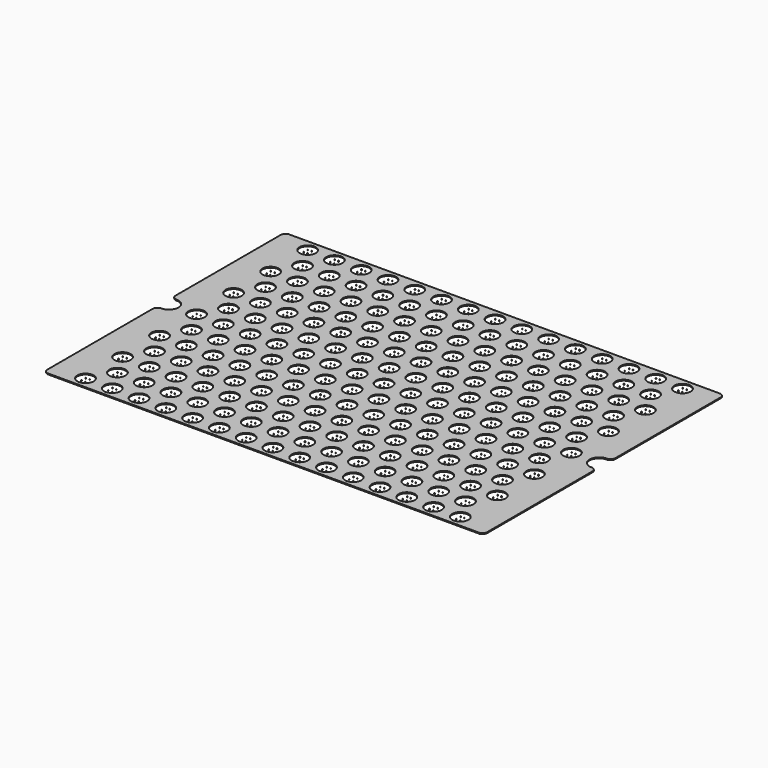
from build123d import *

# Parameters (mm, degrees)
F0_R     = 8.5
F1_DEPTH = 1
F2_R     = 0.25
F3_DEPTH = 1


with BuildPart() as f1:
    # F0 (on Top) → F1 (new body)
    with BuildSketch(Plane.XY):
        with BuildLine():
            Line((225, 157.5), (-225, 157.5))
            ThreePointArc((-225, 157.5), (-228.5355339059, 156.0355339059), (-230, 152.5))
            Line((-230, 152.5), (-230, 15))
            ThreePointArc((-230, 15), (-228.5355339059, 11.4644660941), (-225, 10))
            ThreePointArc((-225, 10), (-215, 0), (-225, -10))
            ThreePointArc((-225, -10), (-228.5355339059, -11.4644660941), (-230, -15))
            Line((-230, -15), (-230, -152.5))
            ThreePointArc((-230, -152.5), (-228.5355339059, -156.0355339059), (-225, -157.5))
            Line((-225, -157.5), (225, -157.5))
            ThreePointArc((225, -157.5), (228.5355339059, -156.0355339059), (230, -152.5))
            Line((230, -152.5), (230, -15))
            ThreePointArc((230, -15), (228.5355339059, -11.4644660941), (225, -10))
            ThreePointArc((225, -10), (215, 0), (225, 10))
            ThreePointArc((225, 10), (228.5355339059, 11.4644660941), (230, 15))
            Line((230, 15), (230, 152.5))
            ThreePointArc((230, 152.5), (228.5355339059, 156.0355339059), (225, 157.5))
        make_face()
        with Locations((-196, -145.2)):
            Circle(F0_R, mode=Mode.SUBTRACT)
        with Locations((-182, -121)):
            Circle(F0_R, mode=Mode.SUBTRACT)
        with Locations((-168, -145.2)):
            Circle(F0_R, mode=Mode.SUBTRACT)
        with Locations((-140, -145.2)):
            Circle(F0_R, mode=Mode.SUBTRACT)
        with Locations((-154, -121)):
            Circle(F0_R, mode=Mode.SUBTRACT)
        with Locations((-126, -121)):
            Circle(F0_R, mode=Mode.SUBTRACT)
        with Locations((-196, -96.8)):
            Circle(F0_R, mode=Mode.SUBTRACT)
        with Locations((-168, -96.8)):
            Circle(F0_R, mode=Mode.SUBTRACT)
        with Locations((-140, -96.8)):
            Circle(F0_R, mode=Mode.SUBTRACT)
        with Locations((-112, -145.2)):
            Circle(F0_R, mode=Mode.SUBTRACT)
        with Locations((-84, -145.2)):
            Circle(F0_R, mode=Mode.SUBTRACT)
        with Locations((-98, -121)):
            Circle(F0_R, mode=Mode.SUBTRACT)
        with Locations((-70, -121)):
            Circle(F0_R, mode=Mode.SUBTRACT)
        with Locations((-56, -145.2)):
            Circle(F0_R, mode=Mode.SUBTRACT)
        with Locations((-28, -145.2)):
            Circle(F0_R, mode=Mode.SUBTRACT)
        with Locations((-42, -121)):
            Circle(F0_R, mode=Mode.SUBTRACT)
        with Locations((-14, -121)):
            Circle(F0_R, mode=Mode.SUBTRACT)
        with Locations((-112, -96.8)):
            Circle(F0_R, mode=Mode.SUBTRACT)
        with Locations((-84, -96.8)):
            Circle(F0_R, mode=Mode.SUBTRACT)
        with Locations((-56, -96.8)):
            Circle(F0_R, mode=Mode.SUBTRACT)
        with Locations((-28, -96.8)):
            Circle(F0_R, mode=Mode.SUBTRACT)
        with Locations((-182, -72.6)):
            Circle(F0_R, mode=Mode.SUBTRACT)
        with Locations((-196, -48.4)):
            Circle(F0_R, mode=Mode.SUBTRACT)
        with Locations((-154, -72.6)):
            Circle(F0_R, mode=Mode.SUBTRACT)
        with Locations((-126, -72.6)):
            Circle(F0_R, mode=Mode.SUBTRACT)
        with Locations((-168, -48.4)):
            Circle(F0_R, mode=Mode.SUBTRACT)
        with Locations((-140, -48.4)):
            Circle(F0_R, mode=Mode.SUBTRACT)
        with Locations((-182, -24.2)):
            Circle(F0_R, mode=Mode.SUBTRACT)
        with Locations((-154, -24.2)):
            Circle(F0_R, mode=Mode.SUBTRACT)
        with Locations((-126, -24.2)):
            Circle(F0_R, mode=Mode.SUBTRACT)
        with Locations((-98, -72.6)):
            Circle(F0_R, mode=Mode.SUBTRACT)
        with Locations((-70, -72.6)):
            Circle(F0_R, mode=Mode.SUBTRACT)
        with Locations((-112, -48.4)):
            Circle(F0_R, mode=Mode.SUBTRACT)
        with Locations((-84, -48.4)):
            Circle(F0_R, mode=Mode.SUBTRACT)
        with Locations((-42, -72.6)):
            Circle(F0_R, mode=Mode.SUBTRACT)
        with Locations((-14, -72.6)):
            Circle(F0_R, mode=Mode.SUBTRACT)
        with Locations((-56, -48.4)):
            Circle(F0_R, mode=Mode.SUBTRACT)
        with Locations((-28, -48.4)):
            Circle(F0_R, mode=Mode.SUBTRACT)
        with Locations((-98, -24.2)):
            Circle(F0_R, mode=Mode.SUBTRACT)
        with Locations((-70, -24.2)):
            Circle(F0_R, mode=Mode.SUBTRACT)
        with Locations((-42, -24.2)):
            Circle(F0_R, mode=Mode.SUBTRACT)
        with Locations((-14, -24.2)):
            Circle(F0_R, mode=Mode.SUBTRACT)
        with Locations((0, -145.2)):
            Circle(F0_R, mode=Mode.SUBTRACT)
        with Locations((28, -145.2)):
            Circle(F0_R, mode=Mode.SUBTRACT)
        with Locations((56, -145.2)):
            Circle(F0_R, mode=Mode.SUBTRACT)
        with Locations((14, -121)):
            Circle(F0_R, mode=Mode.SUBTRACT)
        with Locations((42, -121)):
            Circle(F0_R, mode=Mode.SUBTRACT)
        with Locations((84, -145.2)):
            Circle(F0_R, mode=Mode.SUBTRACT)
        with Locations((112, -145.2)):
            Circle(F0_R, mode=Mode.SUBTRACT)
        with Locations((70, -121)):
            Circle(F0_R, mode=Mode.SUBTRACT)
        with Locations((98, -121)):
            Circle(F0_R, mode=Mode.SUBTRACT)
        with Locations((0, -96.8)):
            Circle(F0_R, mode=Mode.SUBTRACT)
        with Locations((28, -96.8)):
            Circle(F0_R, mode=Mode.SUBTRACT)
        with Locations((56, -96.8)):
            Circle(F0_R, mode=Mode.SUBTRACT)
        with Locations((84, -96.8)):
            Circle(F0_R, mode=Mode.SUBTRACT)
        with Locations((112, -96.8)):
            Circle(F0_R, mode=Mode.SUBTRACT)
        with Locations((140, -145.2)):
            Circle(F0_R, mode=Mode.SUBTRACT)
        with Locations((168, -145.2)):
            Circle(F0_R, mode=Mode.SUBTRACT)
        with Locations((126, -121)):
            Circle(F0_R, mode=Mode.SUBTRACT)
        with Locations((154, -121)):
            Circle(F0_R, mode=Mode.SUBTRACT)
        with Locations((196, -145.2)):
            Circle(F0_R, mode=Mode.SUBTRACT)
        with Locations((182, -121)):
            Circle(F0_R, mode=Mode.SUBTRACT)
        with Locations((140, -96.8)):
            Circle(F0_R, mode=Mode.SUBTRACT)
        with Locations((168, -96.8)):
            Circle(F0_R, mode=Mode.SUBTRACT)
        with Locations((196, -96.8)):
            Circle(F0_R, mode=Mode.SUBTRACT)
        with Locations((14, -72.6)):
            Circle(F0_R, mode=Mode.SUBTRACT)
        with Locations((42, -72.6)):
            Circle(F0_R, mode=Mode.SUBTRACT)
        with Locations((0, -48.4)):
            Circle(F0_R, mode=Mode.SUBTRACT)
        with Locations((28, -48.4)):
            Circle(F0_R, mode=Mode.SUBTRACT)
        with Locations((56, -48.4)):
            Circle(F0_R, mode=Mode.SUBTRACT)
        with Locations((70, -72.6)):
            Circle(F0_R, mode=Mode.SUBTRACT)
        with Locations((98, -72.6)):
            Circle(F0_R, mode=Mode.SUBTRACT)
        with Locations((84, -48.4)):
            Circle(F0_R, mode=Mode.SUBTRACT)
        with Locations((112, -48.4)):
            Circle(F0_R, mode=Mode.SUBTRACT)
        with Locations((14, -24.2)):
            Circle(F0_R, mode=Mode.SUBTRACT)
        with Locations((42, -24.2)):
            Circle(F0_R, mode=Mode.SUBTRACT)
        with Locations((70, -24.2)):
            Circle(F0_R, mode=Mode.SUBTRACT)
        with Locations((98, -24.2)):
            Circle(F0_R, mode=Mode.SUBTRACT)
        with Locations((126, -72.6)):
            Circle(F0_R, mode=Mode.SUBTRACT)
        with Locations((154, -72.6)):
            Circle(F0_R, mode=Mode.SUBTRACT)
        with Locations((140, -48.4)):
            Circle(F0_R, mode=Mode.SUBTRACT)
        with Locations((168, -48.4)):
            Circle(F0_R, mode=Mode.SUBTRACT)
        with Locations((182, -72.6)):
            Circle(F0_R, mode=Mode.SUBTRACT)
        with Locations((196, -48.4)):
            Circle(F0_R, mode=Mode.SUBTRACT)
        with Locations((126, -24.2)):
            Circle(F0_R, mode=Mode.SUBTRACT)
        with Locations((154, -24.2)):
            Circle(F0_R, mode=Mode.SUBTRACT)
        with Locations((182, -24.2)):
            Circle(F0_R, mode=Mode.SUBTRACT)
        with Locations((-196, 0)):
            Circle(F0_R, mode=Mode.SUBTRACT)
        with Locations((-182, 24.2)):
            Circle(F0_R, mode=Mode.SUBTRACT)
        with Locations((-168, 0)):
            Circle(F0_R, mode=Mode.SUBTRACT)
        with Locations((-140, 0)):
            Circle(F0_R, mode=Mode.SUBTRACT)
        with Locations((-154, 24.2)):
            Circle(F0_R, mode=Mode.SUBTRACT)
        with Locations((-126, 24.2)):
            Circle(F0_R, mode=Mode.SUBTRACT)
        with Locations((-196, 48.4)):
            Circle(F0_R, mode=Mode.SUBTRACT)
        with Locations((-182, 72.6)):
            Circle(F0_R, mode=Mode.SUBTRACT)
        with Locations((-168, 48.4)):
            Circle(F0_R, mode=Mode.SUBTRACT)
        with Locations((-140, 48.4)):
            Circle(F0_R, mode=Mode.SUBTRACT)
        with Locations((-154, 72.6)):
            Circle(F0_R, mode=Mode.SUBTRACT)
        with Locations((-126, 72.6)):
            Circle(F0_R, mode=Mode.SUBTRACT)
        with Locations((-112, 0)):
            Circle(F0_R, mode=Mode.SUBTRACT)
        with Locations((-84, 0)):
            Circle(F0_R, mode=Mode.SUBTRACT)
        with Locations((-98, 24.2)):
            Circle(F0_R, mode=Mode.SUBTRACT)
        with Locations((-70, 24.2)):
            Circle(F0_R, mode=Mode.SUBTRACT)
        with Locations((-56, 0)):
            Circle(F0_R, mode=Mode.SUBTRACT)
        with Locations((-28, 0)):
            Circle(F0_R, mode=Mode.SUBTRACT)
        with Locations((-42, 24.2)):
            Circle(F0_R, mode=Mode.SUBTRACT)
        with Locations((-14, 24.2)):
            Circle(F0_R, mode=Mode.SUBTRACT)
        with Locations((-112, 48.4)):
            Circle(F0_R, mode=Mode.SUBTRACT)
        with Locations((-84, 48.4)):
            Circle(F0_R, mode=Mode.SUBTRACT)
        with Locations((-98, 72.6)):
            Circle(F0_R, mode=Mode.SUBTRACT)
        with Locations((-70, 72.6)):
            Circle(F0_R, mode=Mode.SUBTRACT)
        with Locations((-56, 48.4)):
            Circle(F0_R, mode=Mode.SUBTRACT)
        with Locations((-28, 48.4)):
            Circle(F0_R, mode=Mode.SUBTRACT)
        with Locations((-42, 72.6)):
            Circle(F0_R, mode=Mode.SUBTRACT)
        with Locations((-14, 72.6)):
            Circle(F0_R, mode=Mode.SUBTRACT)
        with Locations((-196, 96.8)):
            Circle(F0_R, mode=Mode.SUBTRACT)
        with Locations((-168, 96.8)):
            Circle(F0_R, mode=Mode.SUBTRACT)
        with Locations((-140, 96.8)):
            Circle(F0_R, mode=Mode.SUBTRACT)
        with Locations((-182, 121)):
            Circle(F0_R, mode=Mode.SUBTRACT)
        with Locations((-196, 145.2)):
            Circle(F0_R, mode=Mode.SUBTRACT)
        with Locations((-154, 121)):
            Circle(F0_R, mode=Mode.SUBTRACT)
        with Locations((-126, 121)):
            Circle(F0_R, mode=Mode.SUBTRACT)
        with Locations((-168, 145.2)):
            Circle(F0_R, mode=Mode.SUBTRACT)
        with Locations((-140, 145.2)):
            Circle(F0_R, mode=Mode.SUBTRACT)
        with Locations((-112, 96.8)):
            Circle(F0_R, mode=Mode.SUBTRACT)
        with Locations((-84, 96.8)):
            Circle(F0_R, mode=Mode.SUBTRACT)
        with Locations((-56, 96.8)):
            Circle(F0_R, mode=Mode.SUBTRACT)
        with Locations((-28, 96.8)):
            Circle(F0_R, mode=Mode.SUBTRACT)
        with Locations((-98, 121)):
            Circle(F0_R, mode=Mode.SUBTRACT)
        with Locations((-70, 121)):
            Circle(F0_R, mode=Mode.SUBTRACT)
        with Locations((-112, 145.2)):
            Circle(F0_R, mode=Mode.SUBTRACT)
        with Locations((-84, 145.2)):
            Circle(F0_R, mode=Mode.SUBTRACT)
        with Locations((-42, 121)):
            Circle(F0_R, mode=Mode.SUBTRACT)
        with Locations((-14, 121)):
            Circle(F0_R, mode=Mode.SUBTRACT)
        with Locations((-56, 145.2)):
            Circle(F0_R, mode=Mode.SUBTRACT)
        with Locations((-28, 145.2)):
            Circle(F0_R, mode=Mode.SUBTRACT)
        Circle(F0_R, mode=Mode.SUBTRACT)
        with Locations((28, 0)):
            Circle(F0_R, mode=Mode.SUBTRACT)
        with Locations((56, 0)):
            Circle(F0_R, mode=Mode.SUBTRACT)
        with Locations((14, 24.2)):
            Circle(F0_R, mode=Mode.SUBTRACT)
        with Locations((42, 24.2)):
            Circle(F0_R, mode=Mode.SUBTRACT)
        with Locations((84, 0)):
            Circle(F0_R, mode=Mode.SUBTRACT)
        with Locations((112, 0)):
            Circle(F0_R, mode=Mode.SUBTRACT)
        with Locations((70, 24.2)):
            Circle(F0_R, mode=Mode.SUBTRACT)
        with Locations((98, 24.2)):
            Circle(F0_R, mode=Mode.SUBTRACT)
        with Locations((0, 48.4)):
            Circle(F0_R, mode=Mode.SUBTRACT)
        with Locations((28, 48.4)):
            Circle(F0_R, mode=Mode.SUBTRACT)
        with Locations((56, 48.4)):
            Circle(F0_R, mode=Mode.SUBTRACT)
        with Locations((14, 72.6)):
            Circle(F0_R, mode=Mode.SUBTRACT)
        with Locations((42, 72.6)):
            Circle(F0_R, mode=Mode.SUBTRACT)
        with Locations((84, 48.4)):
            Circle(F0_R, mode=Mode.SUBTRACT)
        with Locations((112, 48.4)):
            Circle(F0_R, mode=Mode.SUBTRACT)
        with Locations((70, 72.6)):
            Circle(F0_R, mode=Mode.SUBTRACT)
        with Locations((98, 72.6)):
            Circle(F0_R, mode=Mode.SUBTRACT)
        with Locations((140, 0)):
            Circle(F0_R, mode=Mode.SUBTRACT)
        with Locations((168, 0)):
            Circle(F0_R, mode=Mode.SUBTRACT)
        with Locations((126, 24.2)):
            Circle(F0_R, mode=Mode.SUBTRACT)
        with Locations((154, 24.2)):
            Circle(F0_R, mode=Mode.SUBTRACT)
        with Locations((196, 0)):
            Circle(F0_R, mode=Mode.SUBTRACT)
        with Locations((182, 24.2)):
            Circle(F0_R, mode=Mode.SUBTRACT)
        with Locations((140, 48.4)):
            Circle(F0_R, mode=Mode.SUBTRACT)
        with Locations((168, 48.4)):
            Circle(F0_R, mode=Mode.SUBTRACT)
        with Locations((126, 72.6)):
            Circle(F0_R, mode=Mode.SUBTRACT)
        with Locations((154, 72.6)):
            Circle(F0_R, mode=Mode.SUBTRACT)
        with Locations((196, 48.4)):
            Circle(F0_R, mode=Mode.SUBTRACT)
        with Locations((182, 72.6)):
            Circle(F0_R, mode=Mode.SUBTRACT)
        with Locations((0, 96.8)):
            Circle(F0_R, mode=Mode.SUBTRACT)
        with Locations((28, 96.8)):
            Circle(F0_R, mode=Mode.SUBTRACT)
        with Locations((56, 96.8)):
            Circle(F0_R, mode=Mode.SUBTRACT)
        with Locations((84, 96.8)):
            Circle(F0_R, mode=Mode.SUBTRACT)
        with Locations((112, 96.8)):
            Circle(F0_R, mode=Mode.SUBTRACT)
        with Locations((14, 121)):
            Circle(F0_R, mode=Mode.SUBTRACT)
        with Locations((42, 121)):
            Circle(F0_R, mode=Mode.SUBTRACT)
        with Locations((0, 145.2)):
            Circle(F0_R, mode=Mode.SUBTRACT)
        with Locations((28, 145.2)):
            Circle(F0_R, mode=Mode.SUBTRACT)
        with Locations((56, 145.2)):
            Circle(F0_R, mode=Mode.SUBTRACT)
        with Locations((70, 121)):
            Circle(F0_R, mode=Mode.SUBTRACT)
        with Locations((98, 121)):
            Circle(F0_R, mode=Mode.SUBTRACT)
        with Locations((84, 145.2)):
            Circle(F0_R, mode=Mode.SUBTRACT)
        with Locations((112, 145.2)):
            Circle(F0_R, mode=Mode.SUBTRACT)
        with Locations((140, 96.8)):
            Circle(F0_R, mode=Mode.SUBTRACT)
        with Locations((168, 96.8)):
            Circle(F0_R, mode=Mode.SUBTRACT)
        with Locations((196, 96.8)):
            Circle(F0_R, mode=Mode.SUBTRACT)
        with Locations((126, 121)):
            Circle(F0_R, mode=Mode.SUBTRACT)
        with Locations((154, 121)):
            Circle(F0_R, mode=Mode.SUBTRACT)
        with Locations((140, 145.2)):
            Circle(F0_R, mode=Mode.SUBTRACT)
        with Locations((168, 145.2)):
            Circle(F0_R, mode=Mode.SUBTRACT)
        with Locations((182, 121)):
            Circle(F0_R, mode=Mode.SUBTRACT)
        with Locations((196, 145.2)):
            Circle(F0_R, mode=Mode.SUBTRACT)
    extrude(amount=F1_DEPTH)


with BuildPart() as f3:
    # F2 (on face) → F3 (new body)
    with BuildSketch(Plane(origin=(0, 0, 0), x_dir=(1, 0, 0), z_dir=(0, 0, -1))):
        with Locations((-197.8294125795, -147.8375941515)):
            Circle(F2_R)
        with Locations((-193.8294125795, -147.8375941515)):
            Circle(F2_R)
        with Locations((-197.8294125795, -142.2375941515)):
            Circle(F2_R)
        with Locations((-193.8294125795, -142.2375941515)):
            Circle(F2_R)
        with Locations((-183.8518373966, -123.4969395161)):
            Circle(F2_R)
        with Locations((-179.8518373966, -123.4969395161)):
            Circle(F2_R)
        with Locations((-179.8518373966, -117.8969395161)):
            Circle(F2_R)
        with Locations((-183.8518373966, -117.8969395161)):
            Circle(F2_R)
        with Locations((-197.8294125795, -99.4375941515)):
            Circle(F2_R)
        with Locations((-193.8294125795, -93.8375941515)):
            Circle(F2_R)
        with Locations((-193.8294125795, -99.4375941515)):
            Circle(F2_R)
        with Locations((-197.8294125795, -93.8375941515)):
            Circle(F2_R)
        with Locations((-197.8294125795, -51.0375941515)):
            Circle(F2_R)
        with Locations((-193.8294125795, -45.4375941515)):
            Circle(F2_R)
        with Locations((-193.8294125795, -51.0375941515)):
            Circle(F2_R)
        with Locations((-197.8294125795, -45.4375941515)):
            Circle(F2_R)
        with Locations((-197.8294125795, -2.6375941515)):
            Circle(F2_R)
        with Locations((-193.8294125795, 2.9624058485)):
            Circle(F2_R)
        with Locations((-193.8294125795, -2.6375941515)):
            Circle(F2_R)
        with Locations((-197.8294125795, 2.9624058485)):
            Circle(F2_R)
        with Locations((-197.8294125795, 45.7624058485)):
            Circle(F2_R)
        with Locations((-193.8294125795, 51.3624058485)):
            Circle(F2_R)
        with Locations((-193.8294125795, 45.7624058485)):
            Circle(F2_R)
        with Locations((-197.8294125795, 51.3624058485)):
            Circle(F2_R)
        with Locations((-197.8294125795, 94.1624058485)):
            Circle(F2_R)
        with Locations((-193.8294125795, 99.7624058485)):
            Circle(F2_R)
        with Locations((-193.8294125795, 94.1624058485)):
            Circle(F2_R)
        with Locations((-197.8294125795, 99.7624058485)):
            Circle(F2_R)
        with Locations((-197.8294125795, 142.5624058485)):
            Circle(F2_R)
        with Locations((-193.8294125795, 148.1624058485)):
            Circle(F2_R)
        with Locations((-193.8294125795, 142.5624058485)):
            Circle(F2_R)
        with Locations((-197.8294125795, 148.1624058485)):
            Circle(F2_R)
        with Locations((-169.8294125795, -147.8375941515)):
            Circle(F2_R)
        with Locations((-165.8294125795, -142.2375941515)):
            Circle(F2_R)
        with Locations((-165.8294125795, -147.8375941515)):
            Circle(F2_R)
        with Locations((-169.8294125795, -142.2375941515)):
            Circle(F2_R)
        with Locations((-169.8294125795, -99.4375941515)):
            Circle(F2_R)
        with Locations((-165.8294125795, -93.8375941515)):
            Circle(F2_R)
        with Locations((-165.8294125795, -99.4375941515)):
            Circle(F2_R)
        with Locations((-169.8294125795, -93.8375941515)):
            Circle(F2_R)
        with Locations((-169.8294125795, -51.0375941515)):
            Circle(F2_R)
        with Locations((-165.8294125795, -45.4375941515)):
            Circle(F2_R)
        with Locations((-165.8294125795, -51.0375941515)):
            Circle(F2_R)
        with Locations((-169.8294125795, -45.4375941515)):
            Circle(F2_R)
        with Locations((-169.8294125795, -2.6375941515)):
            Circle(F2_R)
        with Locations((-165.8294125795, 2.9624058485)):
            Circle(F2_R)
        with Locations((-165.8294125795, -2.6375941515)):
            Circle(F2_R)
        with Locations((-169.8294125795, 2.9624058485)):
            Circle(F2_R)
        with Locations((-169.8294125795, 45.7624058485)):
            Circle(F2_R)
        with Locations((-165.8294125795, 51.3624058485)):
            Circle(F2_R)
        with Locations((-165.8294125795, 45.7624058485)):
            Circle(F2_R)
        with Locations((-169.8294125795, 51.3624058485)):
            Circle(F2_R)
        with Locations((-169.8294125795, 94.1624058485)):
            Circle(F2_R)
        with Locations((-165.8294125795, 99.7624058485)):
            Circle(F2_R)
        with Locations((-165.8294125795, 94.1624058485)):
            Circle(F2_R)
        with Locations((-169.8294125795, 99.7624058485)):
            Circle(F2_R)
        with Locations((-169.8294125795, 142.5624058485)):
            Circle(F2_R)
        with Locations((-165.8294125795, 148.1624058485)):
            Circle(F2_R)
        with Locations((-165.8294125795, 142.5624058485)):
            Circle(F2_R)
        with Locations((-169.8294125795, 148.1624058485)):
            Circle(F2_R)
        with Locations((-141.8294125795, -147.8375941515)):
            Circle(F2_R)
        with Locations((-137.8294125795, -142.2375941515)):
            Circle(F2_R)
        with Locations((-137.8294125795, -147.8375941515)):
            Circle(F2_R)
        with Locations((-141.8294125795, -142.2375941515)):
            Circle(F2_R)
        with Locations((-141.8294125795, -99.4375941515)):
            Circle(F2_R)
        with Locations((-137.8294125795, -93.8375941515)):
            Circle(F2_R)
        with Locations((-137.8294125795, -99.4375941515)):
            Circle(F2_R)
        with Locations((-141.8294125795, -93.8375941515)):
            Circle(F2_R)
        with Locations((-141.8294125795, -51.0375941515)):
            Circle(F2_R)
        with Locations((-137.8294125795, -45.4375941515)):
            Circle(F2_R)
        with Locations((-137.8294125795, -51.0375941515)):
            Circle(F2_R)
        with Locations((-141.8294125795, -45.4375941515)):
            Circle(F2_R)
        with Locations((-141.8294125795, -2.6375941515)):
            Circle(F2_R)
        with Locations((-137.8294125795, 2.9624058485)):
            Circle(F2_R)
        with Locations((-137.8294125795, -2.6375941515)):
            Circle(F2_R)
        with Locations((-141.8294125795, 2.9624058485)):
            Circle(F2_R)
        with Locations((-141.8294125795, 45.7624058485)):
            Circle(F2_R)
        with Locations((-137.8294125795, 51.3624058485)):
            Circle(F2_R)
        with Locations((-137.8294125795, 45.7624058485)):
            Circle(F2_R)
        with Locations((-141.8294125795, 51.3624058485)):
            Circle(F2_R)
        with Locations((-141.8294125795, 94.1624058485)):
            Circle(F2_R)
        with Locations((-137.8294125795, 99.7624058485)):
            Circle(F2_R)
        with Locations((-137.8294125795, 94.1624058485)):
            Circle(F2_R)
        with Locations((-141.8294125795, 99.7624058485)):
            Circle(F2_R)
        with Locations((-141.8294125795, 142.5624058485)):
            Circle(F2_R)
        with Locations((-137.8294125795, 148.1624058485)):
            Circle(F2_R)
        with Locations((-137.8294125795, 142.5624058485)):
            Circle(F2_R)
        with Locations((-141.8294125795, 148.1624058485)):
            Circle(F2_R)
        with Locations((-113.8294125795, -147.8375941515)):
            Circle(F2_R)
        with Locations((-109.8294125795, -142.2375941515)):
            Circle(F2_R)
        with Locations((-109.8294125795, -147.8375941515)):
            Circle(F2_R)
        with Locations((-113.8294125795, -142.2375941515)):
            Circle(F2_R)
        with Locations((-113.8294125795, -99.4375941515)):
            Circle(F2_R)
        with Locations((-109.8294125795, -93.8375941515)):
            Circle(F2_R)
        with Locations((-109.8294125795, -99.4375941515)):
            Circle(F2_R)
        with Locations((-113.8294125795, -93.8375941515)):
            Circle(F2_R)
        with Locations((-113.8294125795, -51.0375941515)):
            Circle(F2_R)
        with Locations((-109.8294125795, -45.4375941515)):
            Circle(F2_R)
        with Locations((-109.8294125795, -51.0375941515)):
            Circle(F2_R)
        with Locations((-113.8294125795, -45.4375941515)):
            Circle(F2_R)
        with Locations((-113.8294125795, -2.6375941515)):
            Circle(F2_R)
        with Locations((-109.8294125795, 2.9624058485)):
            Circle(F2_R)
        with Locations((-109.8294125795, -2.6375941515)):
            Circle(F2_R)
        with Locations((-113.8294125795, 2.9624058485)):
            Circle(F2_R)
        with Locations((-113.8294125795, 45.7624058485)):
            Circle(F2_R)
        with Locations((-109.8294125795, 51.3624058485)):
            Circle(F2_R)
        with Locations((-109.8294125795, 45.7624058485)):
            Circle(F2_R)
        with Locations((-113.8294125795, 51.3624058485)):
            Circle(F2_R)
        with Locations((-113.8294125795, 94.1624058485)):
            Circle(F2_R)
        with Locations((-109.8294125795, 99.7624058485)):
            Circle(F2_R)
        with Locations((-109.8294125795, 94.1624058485)):
            Circle(F2_R)
        with Locations((-113.8294125795, 99.7624058485)):
            Circle(F2_R)
        with Locations((-113.8294125795, 142.5624058485)):
            Circle(F2_R)
        with Locations((-109.8294125795, 148.1624058485)):
            Circle(F2_R)
        with Locations((-109.8294125795, 142.5624058485)):
            Circle(F2_R)
        with Locations((-113.8294125795, 148.1624058485)):
            Circle(F2_R)
        with Locations((-85.8294125795, -147.8375941515)):
            Circle(F2_R)
        with Locations((-81.8294125795, -142.2375941515)):
            Circle(F2_R)
        with Locations((-81.8294125795, -147.8375941515)):
            Circle(F2_R)
        with Locations((-85.8294125795, -142.2375941515)):
            Circle(F2_R)
        with Locations((-85.8294125795, -99.4375941515)):
            Circle(F2_R)
        with Locations((-81.8294125795, -93.8375941515)):
            Circle(F2_R)
        with Locations((-81.8294125795, -99.4375941515)):
            Circle(F2_R)
        with Locations((-85.8294125795, -93.8375941515)):
            Circle(F2_R)
        with Locations((-85.8294125795, -51.0375941515)):
            Circle(F2_R)
        with Locations((-81.8294125795, -45.4375941515)):
            Circle(F2_R)
        with Locations((-81.8294125795, -51.0375941515)):
            Circle(F2_R)
        with Locations((-85.8294125795, -45.4375941515)):
            Circle(F2_R)
        with Locations((-85.8294125795, -2.6375941515)):
            Circle(F2_R)
        with Locations((-81.8294125795, 2.9624058485)):
            Circle(F2_R)
        with Locations((-81.8294125795, -2.6375941515)):
            Circle(F2_R)
        with Locations((-85.8294125795, 2.9624058485)):
            Circle(F2_R)
        with Locations((-85.8294125795, 45.7624058485)):
            Circle(F2_R)
        with Locations((-81.8294125795, 51.3624058485)):
            Circle(F2_R)
        with Locations((-81.8294125795, 45.7624058485)):
            Circle(F2_R)
        with Locations((-85.8294125795, 51.3624058485)):
            Circle(F2_R)
        with Locations((-85.8294125795, 94.1624058485)):
            Circle(F2_R)
        with Locations((-81.8294125795, 99.7624058485)):
            Circle(F2_R)
        with Locations((-81.8294125795, 94.1624058485)):
            Circle(F2_R)
        with Locations((-85.8294125795, 99.7624058485)):
            Circle(F2_R)
        with Locations((-85.8294125795, 142.5624058485)):
            Circle(F2_R)
        with Locations((-81.8294125795, 148.1624058485)):
            Circle(F2_R)
        with Locations((-81.8294125795, 142.5624058485)):
            Circle(F2_R)
        with Locations((-85.8294125795, 148.1624058485)):
            Circle(F2_R)
        with Locations((-57.8294125795, -147.8375941515)):
            Circle(F2_R)
        with Locations((-53.8294125795, -142.2375941515)):
            Circle(F2_R)
        with Locations((-53.8294125795, -147.8375941515)):
            Circle(F2_R)
        with Locations((-57.8294125795, -142.2375941515)):
            Circle(F2_R)
        with Locations((-57.8294125795, -99.4375941515)):
            Circle(F2_R)
        with Locations((-53.8294125795, -93.8375941515)):
            Circle(F2_R)
        with Locations((-53.8294125795, -99.4375941515)):
            Circle(F2_R)
        with Locations((-57.8294125795, -93.8375941515)):
            Circle(F2_R)
        with Locations((-57.8294125795, -51.0375941515)):
            Circle(F2_R)
        with Locations((-53.8294125795, -45.4375941515)):
            Circle(F2_R)
        with Locations((-53.8294125795, -51.0375941515)):
            Circle(F2_R)
        with Locations((-57.8294125795, -45.4375941515)):
            Circle(F2_R)
        with Locations((-57.8294125795, -2.6375941515)):
            Circle(F2_R)
        with Locations((-53.8294125795, 2.9624058485)):
            Circle(F2_R)
        with Locations((-53.8294125795, -2.6375941515)):
            Circle(F2_R)
        with Locations((-57.8294125795, 2.9624058485)):
            Circle(F2_R)
        with Locations((-57.8294125795, 45.7624058485)):
            Circle(F2_R)
        with Locations((-53.8294125795, 51.3624058485)):
            Circle(F2_R)
        with Locations((-53.8294125795, 45.7624058485)):
            Circle(F2_R)
        with Locations((-57.8294125795, 51.3624058485)):
            Circle(F2_R)
        with Locations((-57.8294125795, 94.1624058485)):
            Circle(F2_R)
        with Locations((-53.8294125795, 99.7624058485)):
            Circle(F2_R)
        with Locations((-53.8294125795, 94.1624058485)):
            Circle(F2_R)
        with Locations((-57.8294125795, 99.7624058485)):
            Circle(F2_R)
        with Locations((-57.8294125795, 142.5624058485)):
            Circle(F2_R)
        with Locations((-53.8294125795, 148.1624058485)):
            Circle(F2_R)
        with Locations((-53.8294125795, 142.5624058485)):
            Circle(F2_R)
        with Locations((-57.8294125795, 148.1624058485)):
            Circle(F2_R)
        with Locations((-29.8294125795, -147.8375941515)):
            Circle(F2_R)
        with Locations((-25.8294125795, -142.2375941515)):
            Circle(F2_R)
        with Locations((-25.8294125795, -147.8375941515)):
            Circle(F2_R)
        with Locations((-29.8294125795, -142.2375941515)):
            Circle(F2_R)
        with Locations((-29.8294125795, -99.4375941515)):
            Circle(F2_R)
        with Locations((-25.8294125795, -93.8375941515)):
            Circle(F2_R)
        with Locations((-25.8294125795, -99.4375941515)):
            Circle(F2_R)
        with Locations((-29.8294125795, -93.8375941515)):
            Circle(F2_R)
        with Locations((-29.8294125795, -51.0375941515)):
            Circle(F2_R)
        with Locations((-25.8294125795, -45.4375941515)):
            Circle(F2_R)
        with Locations((-25.8294125795, -51.0375941515)):
            Circle(F2_R)
        with Locations((-29.8294125795, -45.4375941515)):
            Circle(F2_R)
        with Locations((-29.8294125795, -2.6375941515)):
            Circle(F2_R)
        with Locations((-25.8294125795, 2.9624058485)):
            Circle(F2_R)
        with Locations((-25.8294125795, -2.6375941515)):
            Circle(F2_R)
        with Locations((-29.8294125795, 2.9624058485)):
            Circle(F2_R)
        with Locations((-29.8294125795, 45.7624058485)):
            Circle(F2_R)
        with Locations((-25.8294125795, 51.3624058485)):
            Circle(F2_R)
        with Locations((-25.8294125795, 45.7624058485)):
            Circle(F2_R)
        with Locations((-29.8294125795, 51.3624058485)):
            Circle(F2_R)
        with Locations((-29.8294125795, 94.1624058485)):
            Circle(F2_R)
        with Locations((-25.8294125795, 99.7624058485)):
            Circle(F2_R)
        with Locations((-25.8294125795, 94.1624058485)):
            Circle(F2_R)
        with Locations((-29.8294125795, 99.7624058485)):
            Circle(F2_R)
        with Locations((-29.8294125795, 142.5624058485)):
            Circle(F2_R)
        with Locations((-25.8294125795, 148.1624058485)):
            Circle(F2_R)
        with Locations((-25.8294125795, 142.5624058485)):
            Circle(F2_R)
        with Locations((-29.8294125795, 148.1624058485)):
            Circle(F2_R)
        with Locations((-1.8294125795, -147.8375941515)):
            Circle(F2_R)
        with Locations((2.1705874205, -142.2375941515)):
            Circle(F2_R)
        with Locations((2.1705874205, -147.8375941515)):
            Circle(F2_R)
        with Locations((-1.8294125795, -142.2375941515)):
            Circle(F2_R)
        with Locations((-1.8294125795, -99.4375941515)):
            Circle(F2_R)
        with Locations((2.1705874205, -93.8375941515)):
            Circle(F2_R)
        with Locations((2.1705874205, -99.4375941515)):
            Circle(F2_R)
        with Locations((-1.8294125795, -93.8375941515)):
            Circle(F2_R)
        with Locations((-1.8294125795, -51.0375941515)):
            Circle(F2_R)
        with Locations((2.1705874205, -45.4375941515)):
            Circle(F2_R)
        with Locations((2.1705874205, -51.0375941515)):
            Circle(F2_R)
        with Locations((-1.8294125795, -45.4375941515)):
            Circle(F2_R)
        with Locations((-1.8294125795, -2.6375941515)):
            Circle(F2_R)
        with Locations((2.1705874205, 2.9624058485)):
            Circle(F2_R)
        with Locations((2.1705874205, -2.6375941515)):
            Circle(F2_R)
        with Locations((-1.8294125795, 2.9624058485)):
            Circle(F2_R)
        with Locations((-1.8294125795, 45.7624058485)):
            Circle(F2_R)
        with Locations((2.1705874205, 51.3624058485)):
            Circle(F2_R)
        with Locations((2.1705874205, 45.7624058485)):
            Circle(F2_R)
        with Locations((-1.8294125795, 51.3624058485)):
            Circle(F2_R)
        with Locations((-1.8294125795, 94.1624058485)):
            Circle(F2_R)
        with Locations((2.1705874205, 99.7624058485)):
            Circle(F2_R)
        with Locations((2.1705874205, 94.1624058485)):
            Circle(F2_R)
        with Locations((-1.8294125795, 99.7624058485)):
            Circle(F2_R)
        with Locations((-1.8294125795, 142.5624058485)):
            Circle(F2_R)
        with Locations((2.1705874205, 148.1624058485)):
            Circle(F2_R)
        with Locations((2.1705874205, 142.5624058485)):
            Circle(F2_R)
        with Locations((-1.8294125795, 148.1624058485)):
            Circle(F2_R)
        with Locations((26.1705874205, -147.8375941515)):
            Circle(F2_R)
        with Locations((30.1705874205, -142.2375941515)):
            Circle(F2_R)
        with Locations((30.1705874205, -147.8375941515)):
            Circle(F2_R)
        with Locations((26.1705874205, -142.2375941515)):
            Circle(F2_R)
        with Locations((26.1705874205, -99.4375941515)):
            Circle(F2_R)
        with Locations((30.1705874205, -93.8375941515)):
            Circle(F2_R)
        with Locations((30.1705874205, -99.4375941515)):
            Circle(F2_R)
        with Locations((26.1705874205, -93.8375941515)):
            Circle(F2_R)
        with Locations((26.1705874205, -51.0375941515)):
            Circle(F2_R)
        with Locations((30.1705874205, -45.4375941515)):
            Circle(F2_R)
        with Locations((30.1705874205, -51.0375941515)):
            Circle(F2_R)
        with Locations((26.1705874205, -45.4375941515)):
            Circle(F2_R)
        with Locations((26.1705874205, -2.6375941515)):
            Circle(F2_R)
        with Locations((30.1705874205, 2.9624058485)):
            Circle(F2_R)
        with Locations((30.1705874205, -2.6375941515)):
            Circle(F2_R)
        with Locations((26.1705874205, 2.9624058485)):
            Circle(F2_R)
        with Locations((26.1705874205, 45.7624058485)):
            Circle(F2_R)
        with Locations((30.1705874205, 51.3624058485)):
            Circle(F2_R)
        with Locations((30.1705874205, 45.7624058485)):
            Circle(F2_R)
        with Locations((26.1705874205, 51.3624058485)):
            Circle(F2_R)
        with Locations((26.1705874205, 94.1624058485)):
            Circle(F2_R)
        with Locations((30.1705874205, 99.7624058485)):
            Circle(F2_R)
        with Locations((30.1705874205, 94.1624058485)):
            Circle(F2_R)
        with Locations((26.1705874205, 99.7624058485)):
            Circle(F2_R)
        with Locations((26.1705874205, 142.5624058485)):
            Circle(F2_R)
        with Locations((30.1705874205, 148.1624058485)):
            Circle(F2_R)
        with Locations((30.1705874205, 142.5624058485)):
            Circle(F2_R)
        with Locations((26.1705874205, 148.1624058485)):
            Circle(F2_R)
        with Locations((54.1705874205, -147.8375941515)):
            Circle(F2_R)
        with Locations((58.1705874205, -142.2375941515)):
            Circle(F2_R)
        with Locations((58.1705874205, -147.8375941515)):
            Circle(F2_R)
        with Locations((54.1705874205, -142.2375941515)):
            Circle(F2_R)
        with Locations((54.1705874205, -99.4375941515)):
            Circle(F2_R)
        with Locations((58.1705874205, -93.8375941515)):
            Circle(F2_R)
        with Locations((58.1705874205, -99.4375941515)):
            Circle(F2_R)
        with Locations((54.1705874205, -93.8375941515)):
            Circle(F2_R)
        with Locations((54.1705874205, -51.0375941515)):
            Circle(F2_R)
        with Locations((58.1705874205, -45.4375941515)):
            Circle(F2_R)
        with Locations((58.1705874205, -51.0375941515)):
            Circle(F2_R)
        with Locations((54.1705874205, -45.4375941515)):
            Circle(F2_R)
        with Locations((54.1705874205, -2.6375941515)):
            Circle(F2_R)
        with Locations((58.1705874205, 2.9624058485)):
            Circle(F2_R)
        with Locations((58.1705874205, -2.6375941515)):
            Circle(F2_R)
        with Locations((54.1705874205, 2.9624058485)):
            Circle(F2_R)
        with Locations((54.1705874205, 45.7624058485)):
            Circle(F2_R)
        with Locations((58.1705874205, 51.3624058485)):
            Circle(F2_R)
        with Locations((58.1705874205, 45.7624058485)):
            Circle(F2_R)
        with Locations((54.1705874205, 51.3624058485)):
            Circle(F2_R)
        with Locations((54.1705874205, 94.1624058485)):
            Circle(F2_R)
        with Locations((58.1705874205, 99.7624058485)):
            Circle(F2_R)
        with Locations((58.1705874205, 94.1624058485)):
            Circle(F2_R)
        with Locations((54.1705874205, 99.7624058485)):
            Circle(F2_R)
        with Locations((54.1705874205, 142.5624058485)):
            Circle(F2_R)
        with Locations((58.1705874205, 148.1624058485)):
            Circle(F2_R)
        with Locations((58.1705874205, 142.5624058485)):
            Circle(F2_R)
        with Locations((54.1705874205, 148.1624058485)):
            Circle(F2_R)
        with Locations((82.1705874205, -147.8375941515)):
            Circle(F2_R)
        with Locations((86.1705874205, -142.2375941515)):
            Circle(F2_R)
        with Locations((86.1705874205, -147.8375941515)):
            Circle(F2_R)
        with Locations((82.1705874205, -142.2375941515)):
            Circle(F2_R)
        with Locations((82.1705874205, -99.4375941515)):
            Circle(F2_R)
        with Locations((86.1705874205, -93.8375941515)):
            Circle(F2_R)
        with Locations((86.1705874205, -99.4375941515)):
            Circle(F2_R)
        with Locations((82.1705874205, -93.8375941515)):
            Circle(F2_R)
        with Locations((82.1705874205, -51.0375941515)):
            Circle(F2_R)
        with Locations((86.1705874205, -45.4375941515)):
            Circle(F2_R)
        with Locations((86.1705874205, -51.0375941515)):
            Circle(F2_R)
        with Locations((82.1705874205, -45.4375941515)):
            Circle(F2_R)
        with Locations((82.1705874205, -2.6375941515)):
            Circle(F2_R)
        with Locations((86.1705874205, 2.9624058485)):
            Circle(F2_R)
        with Locations((86.1705874205, -2.6375941515)):
            Circle(F2_R)
        with Locations((82.1705874205, 2.9624058485)):
            Circle(F2_R)
        with Locations((82.1705874205, 45.7624058485)):
            Circle(F2_R)
        with Locations((86.1705874205, 51.3624058485)):
            Circle(F2_R)
        with Locations((86.1705874205, 45.7624058485)):
            Circle(F2_R)
        with Locations((82.1705874205, 51.3624058485)):
            Circle(F2_R)
        with Locations((82.1705874205, 94.1624058485)):
            Circle(F2_R)
        with Locations((86.1705874205, 99.7624058485)):
            Circle(F2_R)
        with Locations((86.1705874205, 94.1624058485)):
            Circle(F2_R)
        with Locations((82.1705874205, 99.7624058485)):
            Circle(F2_R)
        with Locations((82.1705874205, 142.5624058485)):
            Circle(F2_R)
        with Locations((86.1705874205, 148.1624058485)):
            Circle(F2_R)
        with Locations((86.1705874205, 142.5624058485)):
            Circle(F2_R)
        with Locations((82.1705874205, 148.1624058485)):
            Circle(F2_R)
        with Locations((110.1705874205, -147.8375941515)):
            Circle(F2_R)
        with Locations((114.1705874205, -142.2375941515)):
            Circle(F2_R)
        with Locations((114.1705874205, -147.8375941515)):
            Circle(F2_R)
        with Locations((110.1705874205, -142.2375941515)):
            Circle(F2_R)
        with Locations((110.1705874205, -99.4375941515)):
            Circle(F2_R)
        with Locations((114.1705874205, -93.8375941515)):
            Circle(F2_R)
        with Locations((114.1705874205, -99.4375941515)):
            Circle(F2_R)
        with Locations((110.1705874205, -93.8375941515)):
            Circle(F2_R)
        with Locations((110.1705874205, -51.0375941515)):
            Circle(F2_R)
        with Locations((114.1705874205, -45.4375941515)):
            Circle(F2_R)
        with Locations((114.1705874205, -51.0375941515)):
            Circle(F2_R)
        with Locations((110.1705874205, -45.4375941515)):
            Circle(F2_R)
        with Locations((110.1705874205, -2.6375941515)):
            Circle(F2_R)
        with Locations((114.1705874205, 2.9624058485)):
            Circle(F2_R)
        with Locations((114.1705874205, -2.6375941515)):
            Circle(F2_R)
        with Locations((110.1705874205, 2.9624058485)):
            Circle(F2_R)
        with Locations((110.1705874205, 45.7624058485)):
            Circle(F2_R)
        with Locations((114.1705874205, 51.3624058485)):
            Circle(F2_R)
        with Locations((114.1705874205, 45.7624058485)):
            Circle(F2_R)
        with Locations((110.1705874205, 51.3624058485)):
            Circle(F2_R)
        with Locations((110.1705874205, 94.1624058485)):
            Circle(F2_R)
        with Locations((114.1705874205, 99.7624058485)):
            Circle(F2_R)
        with Locations((114.1705874205, 94.1624058485)):
            Circle(F2_R)
        with Locations((110.1705874205, 99.7624058485)):
            Circle(F2_R)
        with Locations((110.1705874205, 142.5624058485)):
            Circle(F2_R)
        with Locations((114.1705874205, 148.1624058485)):
            Circle(F2_R)
        with Locations((114.1705874205, 142.5624058485)):
            Circle(F2_R)
        with Locations((110.1705874205, 148.1624058485)):
            Circle(F2_R)
        with Locations((138.1705874205, -147.8375941515)):
            Circle(F2_R)
        with Locations((142.1705874205, -142.2375941515)):
            Circle(F2_R)
        with Locations((142.1705874205, -147.8375941515)):
            Circle(F2_R)
        with Locations((138.1705874205, -142.2375941515)):
            Circle(F2_R)
        with Locations((138.1705874205, -99.4375941515)):
            Circle(F2_R)
        with Locations((142.1705874205, -93.8375941515)):
            Circle(F2_R)
        with Locations((142.1705874205, -99.4375941515)):
            Circle(F2_R)
        with Locations((138.1705874205, -93.8375941515)):
            Circle(F2_R)
        with Locations((138.1705874205, -51.0375941515)):
            Circle(F2_R)
        with Locations((142.1705874205, -45.4375941515)):
            Circle(F2_R)
        with Locations((142.1705874205, -51.0375941515)):
            Circle(F2_R)
        with Locations((138.1705874205, -45.4375941515)):
            Circle(F2_R)
        with Locations((138.1705874205, -2.6375941515)):
            Circle(F2_R)
        with Locations((142.1705874205, 2.9624058485)):
            Circle(F2_R)
        with Locations((142.1705874205, -2.6375941515)):
            Circle(F2_R)
        with Locations((138.1705874205, 2.9624058485)):
            Circle(F2_R)
        with Locations((138.1705874205, 45.7624058485)):
            Circle(F2_R)
        with Locations((142.1705874205, 51.3624058485)):
            Circle(F2_R)
        with Locations((142.1705874205, 45.7624058485)):
            Circle(F2_R)
        with Locations((138.1705874205, 51.3624058485)):
            Circle(F2_R)
        with Locations((138.1705874205, 94.1624058485)):
            Circle(F2_R)
        with Locations((142.1705874205, 99.7624058485)):
            Circle(F2_R)
        with Locations((142.1705874205, 94.1624058485)):
            Circle(F2_R)
        with Locations((138.1705874205, 99.7624058485)):
            Circle(F2_R)
        with Locations((138.1705874205, 142.5624058485)):
            Circle(F2_R)
        with Locations((142.1705874205, 148.1624058485)):
            Circle(F2_R)
        with Locations((142.1705874205, 142.5624058485)):
            Circle(F2_R)
        with Locations((138.1705874205, 148.1624058485)):
            Circle(F2_R)
        with Locations((166.1705874205, -147.8375941515)):
            Circle(F2_R)
        with Locations((170.1705874205, -142.2375941515)):
            Circle(F2_R)
        with Locations((170.1705874205, -147.8375941515)):
            Circle(F2_R)
        with Locations((166.1705874205, -142.2375941515)):
            Circle(F2_R)
        with Locations((166.1705874205, -99.4375941515)):
            Circle(F2_R)
        with Locations((170.1705874205, -93.8375941515)):
            Circle(F2_R)
        with Locations((170.1705874205, -99.4375941515)):
            Circle(F2_R)
        with Locations((166.1705874205, -93.8375941515)):
            Circle(F2_R)
        with Locations((166.1705874205, -51.0375941515)):
            Circle(F2_R)
        with Locations((170.1705874205, -45.4375941515)):
            Circle(F2_R)
        with Locations((170.1705874205, -51.0375941515)):
            Circle(F2_R)
        with Locations((166.1705874205, -45.4375941515)):
            Circle(F2_R)
        with Locations((166.1705874205, -2.6375941515)):
            Circle(F2_R)
        with Locations((170.1705874205, 2.9624058485)):
            Circle(F2_R)
        with Locations((170.1705874205, -2.6375941515)):
            Circle(F2_R)
        with Locations((166.1705874205, 2.9624058485)):
            Circle(F2_R)
        with Locations((166.1705874205, 45.7624058485)):
            Circle(F2_R)
        with Locations((170.1705874205, 51.3624058485)):
            Circle(F2_R)
        with Locations((170.1705874205, 45.7624058485)):
            Circle(F2_R)
        with Locations((166.1705874205, 51.3624058485)):
            Circle(F2_R)
        with Locations((166.1705874205, 94.1624058485)):
            Circle(F2_R)
        with Locations((170.1705874205, 99.7624058485)):
            Circle(F2_R)
        with Locations((170.1705874205, 94.1624058485)):
            Circle(F2_R)
        with Locations((166.1705874205, 99.7624058485)):
            Circle(F2_R)
        with Locations((166.1705874205, 142.5624058485)):
            Circle(F2_R)
        with Locations((170.1705874205, 148.1624058485)):
            Circle(F2_R)
        with Locations((170.1705874205, 142.5624058485)):
            Circle(F2_R)
        with Locations((166.1705874205, 148.1624058485)):
            Circle(F2_R)
        with Locations((194.1705874205, -147.8375941515)):
            Circle(F2_R)
        with Locations((198.1705874205, -142.2375941515)):
            Circle(F2_R)
        with Locations((198.1705874205, -147.8375941515)):
            Circle(F2_R)
        with Locations((194.1705874205, -142.2375941515)):
            Circle(F2_R)
        with Locations((194.1705874205, -99.4375941515)):
            Circle(F2_R)
        with Locations((198.1705874205, -93.8375941515)):
            Circle(F2_R)
        with Locations((198.1705874205, -99.4375941515)):
            Circle(F2_R)
        with Locations((194.1705874205, -93.8375941515)):
            Circle(F2_R)
        with Locations((194.1705874205, -51.0375941515)):
            Circle(F2_R)
        with Locations((198.1705874205, -45.4375941515)):
            Circle(F2_R)
        with Locations((198.1705874205, -51.0375941515)):
            Circle(F2_R)
        with Locations((194.1705874205, -45.4375941515)):
            Circle(F2_R)
        with Locations((194.1705874205, -2.6375941515)):
            Circle(F2_R)
        with Locations((198.1705874205, 2.9624058485)):
            Circle(F2_R)
        with Locations((198.1705874205, -2.6375941515)):
            Circle(F2_R)
        with Locations((194.1705874205, 2.9624058485)):
            Circle(F2_R)
        with Locations((194.1705874205, 45.7624058485)):
            Circle(F2_R)
        with Locations((198.1705874205, 51.3624058485)):
            Circle(F2_R)
        with Locations((198.1705874205, 45.7624058485)):
            Circle(F2_R)
        with Locations((194.1705874205, 51.3624058485)):
            Circle(F2_R)
        with Locations((194.1705874205, 94.1624058485)):
            Circle(F2_R)
        with Locations((198.1705874205, 99.7624058485)):
            Circle(F2_R)
        with Locations((198.1705874205, 94.1624058485)):
            Circle(F2_R)
        with Locations((194.1705874205, 99.7624058485)):
            Circle(F2_R)
        with Locations((194.1705874205, 142.5624058485)):
            Circle(F2_R)
        with Locations((198.1705874205, 148.1624058485)):
            Circle(F2_R)
        with Locations((198.1705874205, 142.5624058485)):
            Circle(F2_R)
        with Locations((194.1705874205, 148.1624058485)):
            Circle(F2_R)
        with Locations((-183.8518373966, -69.4969395161)):
            Circle(F2_R)
        with Locations((-179.8518373966, -69.4969395161)):
            Circle(F2_R)
        with Locations((-183.8518373966, -75.0969395161)):
            Circle(F2_R)
        with Locations((-179.8518373966, -75.0969395161)):
            Circle(F2_R)
        with Locations((-183.8518373966, -21.0969395161)):
            Circle(F2_R)
        with Locations((-179.8518373966, -21.0969395161)):
            Circle(F2_R)
        with Locations((-183.8518373966, -26.6969395161)):
            Circle(F2_R)
        with Locations((-179.8518373966, -26.6969395161)):
            Circle(F2_R)
        with Locations((-183.8518373966, 27.3030604839)):
            Circle(F2_R)
        with Locations((-179.8518373966, 27.3030604839)):
            Circle(F2_R)
        with Locations((-183.8518373966, 21.7030604839)):
            Circle(F2_R)
        with Locations((-179.8518373966, 21.7030604839)):
            Circle(F2_R)
        with Locations((-183.8518373966, 75.7030604839)):
            Circle(F2_R)
        with Locations((-179.8518373966, 75.7030604839)):
            Circle(F2_R)
        with Locations((-183.8518373966, 70.1030604839)):
            Circle(F2_R)
        with Locations((-179.8518373966, 70.1030604839)):
            Circle(F2_R)
        with Locations((-183.8518373966, 124.1030604839)):
            Circle(F2_R)
        with Locations((-179.8518373966, 124.1030604839)):
            Circle(F2_R)
        with Locations((-183.8518373966, 118.5030604839)):
            Circle(F2_R)
        with Locations((-179.8518373966, 118.5030604839)):
            Circle(F2_R)
        with Locations((-155.8518373966, -117.8969395161)):
            Circle(F2_R)
        with Locations((-151.8518373966, -117.8969395161)):
            Circle(F2_R)
        with Locations((-155.8518373966, -123.4969395161)):
            Circle(F2_R)
        with Locations((-151.8518373966, -123.4969395161)):
            Circle(F2_R)
        with Locations((-155.8518373966, -69.4969395161)):
            Circle(F2_R)
        with Locations((-151.8518373966, -69.4969395161)):
            Circle(F2_R)
        with Locations((-155.8518373966, -75.0969395161)):
            Circle(F2_R)
        with Locations((-151.8518373966, -75.0969395161)):
            Circle(F2_R)
        with Locations((-155.8518373966, -21.0969395161)):
            Circle(F2_R)
        with Locations((-151.8518373966, -21.0969395161)):
            Circle(F2_R)
        with Locations((-155.8518373966, -26.6969395161)):
            Circle(F2_R)
        with Locations((-151.8518373966, -26.6969395161)):
            Circle(F2_R)
        with Locations((-155.8518373966, 27.3030604839)):
            Circle(F2_R)
        with Locations((-151.8518373966, 27.3030604839)):
            Circle(F2_R)
        with Locations((-155.8518373966, 21.7030604839)):
            Circle(F2_R)
        with Locations((-151.8518373966, 21.7030604839)):
            Circle(F2_R)
        with Locations((-155.8518373966, 75.7030604839)):
            Circle(F2_R)
        with Locations((-151.8518373966, 75.7030604839)):
            Circle(F2_R)
        with Locations((-155.8518373966, 70.1030604839)):
            Circle(F2_R)
        with Locations((-151.8518373966, 70.1030604839)):
            Circle(F2_R)
        with Locations((-155.8518373966, 124.1030604839)):
            Circle(F2_R)
        with Locations((-151.8518373966, 124.1030604839)):
            Circle(F2_R)
        with Locations((-155.8518373966, 118.5030604839)):
            Circle(F2_R)
        with Locations((-151.8518373966, 118.5030604839)):
            Circle(F2_R)
        with Locations((-127.8518373966, -117.8969395161)):
            Circle(F2_R)
        with Locations((-123.8518373966, -117.8969395161)):
            Circle(F2_R)
        with Locations((-127.8518373966, -123.4969395161)):
            Circle(F2_R)
        with Locations((-123.8518373966, -123.4969395161)):
            Circle(F2_R)
        with Locations((-127.8518373966, -69.4969395161)):
            Circle(F2_R)
        with Locations((-123.8518373966, -69.4969395161)):
            Circle(F2_R)
        with Locations((-127.8518373966, -75.0969395161)):
            Circle(F2_R)
        with Locations((-123.8518373966, -75.0969395161)):
            Circle(F2_R)
        with Locations((-127.8518373966, -21.0969395161)):
            Circle(F2_R)
        with Locations((-123.8518373966, -21.0969395161)):
            Circle(F2_R)
        with Locations((-127.8518373966, -26.6969395161)):
            Circle(F2_R)
        with Locations((-123.8518373966, -26.6969395161)):
            Circle(F2_R)
        with Locations((-127.8518373966, 27.3030604839)):
            Circle(F2_R)
        with Locations((-123.8518373966, 27.3030604839)):
            Circle(F2_R)
        with Locations((-127.8518373966, 21.7030604839)):
            Circle(F2_R)
        with Locations((-123.8518373966, 21.7030604839)):
            Circle(F2_R)
        with Locations((-127.8518373966, 75.7030604839)):
            Circle(F2_R)
        with Locations((-123.8518373966, 75.7030604839)):
            Circle(F2_R)
        with Locations((-127.8518373966, 70.1030604839)):
            Circle(F2_R)
        with Locations((-123.8518373966, 70.1030604839)):
            Circle(F2_R)
        with Locations((-127.8518373966, 124.1030604839)):
            Circle(F2_R)
        with Locations((-123.8518373966, 124.1030604839)):
            Circle(F2_R)
        with Locations((-127.8518373966, 118.5030604839)):
            Circle(F2_R)
        with Locations((-123.8518373966, 118.5030604839)):
            Circle(F2_R)
        with Locations((-99.8518373966, -117.8969395161)):
            Circle(F2_R)
        with Locations((-95.8518373966, -117.8969395161)):
            Circle(F2_R)
        with Locations((-99.8518373966, -123.4969395161)):
            Circle(F2_R)
        with Locations((-95.8518373966, -123.4969395161)):
            Circle(F2_R)
        with Locations((-99.8518373966, -69.4969395161)):
            Circle(F2_R)
        with Locations((-95.8518373966, -69.4969395161)):
            Circle(F2_R)
        with Locations((-99.8518373966, -75.0969395161)):
            Circle(F2_R)
        with Locations((-95.8518373966, -75.0969395161)):
            Circle(F2_R)
        with Locations((-99.8518373966, -21.0969395161)):
            Circle(F2_R)
        with Locations((-95.8518373966, -21.0969395161)):
            Circle(F2_R)
        with Locations((-99.8518373966, -26.6969395161)):
            Circle(F2_R)
        with Locations((-95.8518373966, -26.6969395161)):
            Circle(F2_R)
        with Locations((-99.8518373966, 27.3030604839)):
            Circle(F2_R)
        with Locations((-95.8518373966, 27.3030604839)):
            Circle(F2_R)
        with Locations((-99.8518373966, 21.7030604839)):
            Circle(F2_R)
        with Locations((-95.8518373966, 21.7030604839)):
            Circle(F2_R)
        with Locations((-99.8518373966, 75.7030604839)):
            Circle(F2_R)
        with Locations((-95.8518373966, 75.7030604839)):
            Circle(F2_R)
        with Locations((-99.8518373966, 70.1030604839)):
            Circle(F2_R)
        with Locations((-95.8518373966, 70.1030604839)):
            Circle(F2_R)
        with Locations((-99.8518373966, 124.1030604839)):
            Circle(F2_R)
        with Locations((-95.8518373966, 124.1030604839)):
            Circle(F2_R)
        with Locations((-99.8518373966, 118.5030604839)):
            Circle(F2_R)
        with Locations((-95.8518373966, 118.5030604839)):
            Circle(F2_R)
        with Locations((-71.8518373966, -117.8969395161)):
            Circle(F2_R)
        with Locations((-67.8518373966, -117.8969395161)):
            Circle(F2_R)
        with Locations((-71.8518373966, -123.4969395161)):
            Circle(F2_R)
        with Locations((-67.8518373966, -123.4969395161)):
            Circle(F2_R)
        with Locations((-71.8518373966, -69.4969395161)):
            Circle(F2_R)
        with Locations((-67.8518373966, -69.4969395161)):
            Circle(F2_R)
        with Locations((-71.8518373966, -75.0969395161)):
            Circle(F2_R)
        with Locations((-67.8518373966, -75.0969395161)):
            Circle(F2_R)
        with Locations((-71.8518373966, -21.0969395161)):
            Circle(F2_R)
        with Locations((-67.8518373966, -21.0969395161)):
            Circle(F2_R)
        with Locations((-71.8518373966, -26.6969395161)):
            Circle(F2_R)
        with Locations((-67.8518373966, -26.6969395161)):
            Circle(F2_R)
        with Locations((-71.8518373966, 27.3030604839)):
            Circle(F2_R)
        with Locations((-67.8518373966, 27.3030604839)):
            Circle(F2_R)
        with Locations((-71.8518373966, 21.7030604839)):
            Circle(F2_R)
        with Locations((-67.8518373966, 21.7030604839)):
            Circle(F2_R)
        with Locations((-71.8518373966, 75.7030604839)):
            Circle(F2_R)
        with Locations((-67.8518373966, 75.7030604839)):
            Circle(F2_R)
        with Locations((-71.8518373966, 70.1030604839)):
            Circle(F2_R)
        with Locations((-67.8518373966, 70.1030604839)):
            Circle(F2_R)
        with Locations((-71.8518373966, 124.1030604839)):
            Circle(F2_R)
        with Locations((-67.8518373966, 124.1030604839)):
            Circle(F2_R)
        with Locations((-71.8518373966, 118.5030604839)):
            Circle(F2_R)
        with Locations((-67.8518373966, 118.5030604839)):
            Circle(F2_R)
        with Locations((-43.8518373966, -117.8969395161)):
            Circle(F2_R)
        with Locations((-39.8518373966, -117.8969395161)):
            Circle(F2_R)
        with Locations((-43.8518373966, -123.4969395161)):
            Circle(F2_R)
        with Locations((-39.8518373966, -123.4969395161)):
            Circle(F2_R)
        with Locations((-43.8518373966, -69.4969395161)):
            Circle(F2_R)
        with Locations((-39.8518373966, -69.4969395161)):
            Circle(F2_R)
        with Locations((-43.8518373966, -75.0969395161)):
            Circle(F2_R)
        with Locations((-39.8518373966, -75.0969395161)):
            Circle(F2_R)
        with Locations((-43.8518373966, -21.0969395161)):
            Circle(F2_R)
        with Locations((-39.8518373966, -21.0969395161)):
            Circle(F2_R)
        with Locations((-43.8518373966, -26.6969395161)):
            Circle(F2_R)
        with Locations((-39.8518373966, -26.6969395161)):
            Circle(F2_R)
        with Locations((-43.8518373966, 27.3030604839)):
            Circle(F2_R)
        with Locations((-39.8518373966, 27.3030604839)):
            Circle(F2_R)
        with Locations((-43.8518373966, 21.7030604839)):
            Circle(F2_R)
        with Locations((-39.8518373966, 21.7030604839)):
            Circle(F2_R)
        with Locations((-43.8518373966, 75.7030604839)):
            Circle(F2_R)
        with Locations((-39.8518373966, 75.7030604839)):
            Circle(F2_R)
        with Locations((-43.8518373966, 70.1030604839)):
            Circle(F2_R)
        with Locations((-39.8518373966, 70.1030604839)):
            Circle(F2_R)
        with Locations((-43.8518373966, 124.1030604839)):
            Circle(F2_R)
        with Locations((-39.8518373966, 124.1030604839)):
            Circle(F2_R)
        with Locations((-43.8518373966, 118.5030604839)):
            Circle(F2_R)
        with Locations((-39.8518373966, 118.5030604839)):
            Circle(F2_R)
        with Locations((-15.8518373966, -117.8969395161)):
            Circle(F2_R)
        with Locations((-11.8518373966, -117.8969395161)):
            Circle(F2_R)
        with Locations((-15.8518373966, -123.4969395161)):
            Circle(F2_R)
        with Locations((-11.8518373966, -123.4969395161)):
            Circle(F2_R)
        with Locations((-15.8518373966, -69.4969395161)):
            Circle(F2_R)
        with Locations((-11.8518373966, -69.4969395161)):
            Circle(F2_R)
        with Locations((-15.8518373966, -75.0969395161)):
            Circle(F2_R)
        with Locations((-11.8518373966, -75.0969395161)):
            Circle(F2_R)
        with Locations((-15.8518373966, -21.0969395161)):
            Circle(F2_R)
        with Locations((-11.8518373966, -21.0969395161)):
            Circle(F2_R)
        with Locations((-15.8518373966, -26.6969395161)):
            Circle(F2_R)
        with Locations((-11.8518373966, -26.6969395161)):
            Circle(F2_R)
        with Locations((-15.8518373966, 27.3030604839)):
            Circle(F2_R)
        with Locations((-11.8518373966, 27.3030604839)):
            Circle(F2_R)
        with Locations((-15.8518373966, 21.7030604839)):
            Circle(F2_R)
        with Locations((-11.8518373966, 21.7030604839)):
            Circle(F2_R)
        with Locations((-15.8518373966, 75.7030604839)):
            Circle(F2_R)
        with Locations((-11.8518373966, 75.7030604839)):
            Circle(F2_R)
        with Locations((-15.8518373966, 70.1030604839)):
            Circle(F2_R)
        with Locations((-11.8518373966, 70.1030604839)):
            Circle(F2_R)
        with Locations((-15.8518373966, 124.1030604839)):
            Circle(F2_R)
        with Locations((-11.8518373966, 124.1030604839)):
            Circle(F2_R)
        with Locations((-15.8518373966, 118.5030604839)):
            Circle(F2_R)
        with Locations((-11.8518373966, 118.5030604839)):
            Circle(F2_R)
        with Locations((12.1481626034, -117.8969395161)):
            Circle(F2_R)
        with Locations((16.1481626034, -117.8969395161)):
            Circle(F2_R)
        with Locations((12.1481626034, -123.4969395161)):
            Circle(F2_R)
        with Locations((16.1481626034, -123.4969395161)):
            Circle(F2_R)
        with Locations((12.1481626034, -69.4969395161)):
            Circle(F2_R)
        with Locations((16.1481626034, -69.4969395161)):
            Circle(F2_R)
        with Locations((12.1481626034, -75.0969395161)):
            Circle(F2_R)
        with Locations((16.1481626034, -75.0969395161)):
            Circle(F2_R)
        with Locations((12.1481626034, -21.0969395161)):
            Circle(F2_R)
        with Locations((16.1481626034, -21.0969395161)):
            Circle(F2_R)
        with Locations((12.1481626034, -26.6969395161)):
            Circle(F2_R)
        with Locations((16.1481626034, -26.6969395161)):
            Circle(F2_R)
        with Locations((12.1481626034, 27.3030604839)):
            Circle(F2_R)
        with Locations((16.1481626034, 27.3030604839)):
            Circle(F2_R)
        with Locations((12.1481626034, 21.7030604839)):
            Circle(F2_R)
        with Locations((16.1481626034, 21.7030604839)):
            Circle(F2_R)
        with Locations((12.1481626034, 75.7030604839)):
            Circle(F2_R)
        with Locations((16.1481626034, 75.7030604839)):
            Circle(F2_R)
        with Locations((12.1481626034, 70.1030604839)):
            Circle(F2_R)
        with Locations((16.1481626034, 70.1030604839)):
            Circle(F2_R)
        with Locations((12.1481626034, 124.1030604839)):
            Circle(F2_R)
        with Locations((16.1481626034, 124.1030604839)):
            Circle(F2_R)
        with Locations((12.1481626034, 118.5030604839)):
            Circle(F2_R)
        with Locations((16.1481626034, 118.5030604839)):
            Circle(F2_R)
        with Locations((40.1481626034, -117.8969395161)):
            Circle(F2_R)
        with Locations((44.1481626034, -117.8969395161)):
            Circle(F2_R)
        with Locations((40.1481626034, -123.4969395161)):
            Circle(F2_R)
        with Locations((44.1481626034, -123.4969395161)):
            Circle(F2_R)
        with Locations((40.1481626034, -69.4969395161)):
            Circle(F2_R)
        with Locations((44.1481626034, -69.4969395161)):
            Circle(F2_R)
        with Locations((40.1481626034, -75.0969395161)):
            Circle(F2_R)
        with Locations((44.1481626034, -75.0969395161)):
            Circle(F2_R)
        with Locations((40.1481626034, -21.0969395161)):
            Circle(F2_R)
        with Locations((44.1481626034, -21.0969395161)):
            Circle(F2_R)
        with Locations((40.1481626034, -26.6969395161)):
            Circle(F2_R)
        with Locations((44.1481626034, -26.6969395161)):
            Circle(F2_R)
        with Locations((40.1481626034, 27.3030604839)):
            Circle(F2_R)
        with Locations((44.1481626034, 27.3030604839)):
            Circle(F2_R)
        with Locations((40.1481626034, 21.7030604839)):
            Circle(F2_R)
        with Locations((44.1481626034, 21.7030604839)):
            Circle(F2_R)
        with Locations((40.1481626034, 75.7030604839)):
            Circle(F2_R)
        with Locations((44.1481626034, 75.7030604839)):
            Circle(F2_R)
        with Locations((40.1481626034, 70.1030604839)):
            Circle(F2_R)
        with Locations((44.1481626034, 70.1030604839)):
            Circle(F2_R)
        with Locations((40.1481626034, 124.1030604839)):
            Circle(F2_R)
        with Locations((44.1481626034, 124.1030604839)):
            Circle(F2_R)
        with Locations((40.1481626034, 118.5030604839)):
            Circle(F2_R)
        with Locations((44.1481626034, 118.5030604839)):
            Circle(F2_R)
        with Locations((68.1481626034, -117.8969395161)):
            Circle(F2_R)
        with Locations((72.1481626034, -117.8969395161)):
            Circle(F2_R)
        with Locations((68.1481626034, -123.4969395161)):
            Circle(F2_R)
        with Locations((72.1481626034, -123.4969395161)):
            Circle(F2_R)
        with Locations((68.1481626034, -69.4969395161)):
            Circle(F2_R)
        with Locations((72.1481626034, -69.4969395161)):
            Circle(F2_R)
        with Locations((68.1481626034, -75.0969395161)):
            Circle(F2_R)
        with Locations((72.1481626034, -75.0969395161)):
            Circle(F2_R)
        with Locations((68.1481626034, -21.0969395161)):
            Circle(F2_R)
        with Locations((72.1481626034, -21.0969395161)):
            Circle(F2_R)
        with Locations((68.1481626034, -26.6969395161)):
            Circle(F2_R)
        with Locations((72.1481626034, -26.6969395161)):
            Circle(F2_R)
        with Locations((68.1481626034, 27.3030604839)):
            Circle(F2_R)
        with Locations((72.1481626034, 27.3030604839)):
            Circle(F2_R)
        with Locations((68.1481626034, 21.7030604839)):
            Circle(F2_R)
        with Locations((72.1481626034, 21.7030604839)):
            Circle(F2_R)
        with Locations((68.1481626034, 75.7030604839)):
            Circle(F2_R)
        with Locations((72.1481626034, 75.7030604839)):
            Circle(F2_R)
        with Locations((68.1481626034, 70.1030604839)):
            Circle(F2_R)
        with Locations((72.1481626034, 70.1030604839)):
            Circle(F2_R)
        with Locations((68.1481626034, 124.1030604839)):
            Circle(F2_R)
        with Locations((72.1481626034, 124.1030604839)):
            Circle(F2_R)
        with Locations((68.1481626034, 118.5030604839)):
            Circle(F2_R)
        with Locations((72.1481626034, 118.5030604839)):
            Circle(F2_R)
        with Locations((96.1481626034, -117.8969395161)):
            Circle(F2_R)
        with Locations((100.1481626034, -117.8969395161)):
            Circle(F2_R)
        with Locations((96.1481626034, -123.4969395161)):
            Circle(F2_R)
        with Locations((100.1481626034, -123.4969395161)):
            Circle(F2_R)
        with Locations((96.1481626034, -69.4969395161)):
            Circle(F2_R)
        with Locations((100.1481626034, -69.4969395161)):
            Circle(F2_R)
        with Locations((96.1481626034, -75.0969395161)):
            Circle(F2_R)
        with Locations((100.1481626034, -75.0969395161)):
            Circle(F2_R)
        with Locations((96.1481626034, -21.0969395161)):
            Circle(F2_R)
        with Locations((100.1481626034, -21.0969395161)):
            Circle(F2_R)
        with Locations((96.1481626034, -26.6969395161)):
            Circle(F2_R)
        with Locations((100.1481626034, -26.6969395161)):
            Circle(F2_R)
        with Locations((96.1481626034, 27.3030604839)):
            Circle(F2_R)
        with Locations((100.1481626034, 27.3030604839)):
            Circle(F2_R)
        with Locations((96.1481626034, 21.7030604839)):
            Circle(F2_R)
        with Locations((100.1481626034, 21.7030604839)):
            Circle(F2_R)
        with Locations((96.1481626034, 75.7030604839)):
            Circle(F2_R)
        with Locations((100.1481626034, 75.7030604839)):
            Circle(F2_R)
        with Locations((96.1481626034, 70.1030604839)):
            Circle(F2_R)
        with Locations((100.1481626034, 70.1030604839)):
            Circle(F2_R)
        with Locations((96.1481626034, 124.1030604839)):
            Circle(F2_R)
        with Locations((100.1481626034, 124.1030604839)):
            Circle(F2_R)
        with Locations((96.1481626034, 118.5030604839)):
            Circle(F2_R)
        with Locations((100.1481626034, 118.5030604839)):
            Circle(F2_R)
        with Locations((124.1481626034, -117.8969395161)):
            Circle(F2_R)
        with Locations((128.1481626034, -117.8969395161)):
            Circle(F2_R)
        with Locations((124.1481626034, -123.4969395161)):
            Circle(F2_R)
        with Locations((128.1481626034, -123.4969395161)):
            Circle(F2_R)
        with Locations((124.1481626034, -69.4969395161)):
            Circle(F2_R)
        with Locations((128.1481626034, -69.4969395161)):
            Circle(F2_R)
        with Locations((124.1481626034, -75.0969395161)):
            Circle(F2_R)
        with Locations((128.1481626034, -75.0969395161)):
            Circle(F2_R)
        with Locations((124.1481626034, -21.0969395161)):
            Circle(F2_R)
        with Locations((128.1481626034, -21.0969395161)):
            Circle(F2_R)
        with Locations((124.1481626034, -26.6969395161)):
            Circle(F2_R)
        with Locations((128.1481626034, -26.6969395161)):
            Circle(F2_R)
        with Locations((124.1481626034, 27.3030604839)):
            Circle(F2_R)
        with Locations((128.1481626034, 27.3030604839)):
            Circle(F2_R)
        with Locations((124.1481626034, 21.7030604839)):
            Circle(F2_R)
        with Locations((128.1481626034, 21.7030604839)):
            Circle(F2_R)
        with Locations((124.1481626034, 75.7030604839)):
            Circle(F2_R)
        with Locations((128.1481626034, 75.7030604839)):
            Circle(F2_R)
        with Locations((124.1481626034, 70.1030604839)):
            Circle(F2_R)
        with Locations((128.1481626034, 70.1030604839)):
            Circle(F2_R)
        with Locations((124.1481626034, 124.1030604839)):
            Circle(F2_R)
        with Locations((128.1481626034, 124.1030604839)):
            Circle(F2_R)
        with Locations((124.1481626034, 118.5030604839)):
            Circle(F2_R)
        with Locations((128.1481626034, 118.5030604839)):
            Circle(F2_R)
        with Locations((152.1481626034, -117.8969395161)):
            Circle(F2_R)
        with Locations((156.1481626034, -117.8969395161)):
            Circle(F2_R)
        with Locations((152.1481626034, -123.4969395161)):
            Circle(F2_R)
        with Locations((156.1481626034, -123.4969395161)):
            Circle(F2_R)
        with Locations((152.1481626034, -69.4969395161)):
            Circle(F2_R)
        with Locations((156.1481626034, -69.4969395161)):
            Circle(F2_R)
        with Locations((152.1481626034, -75.0969395161)):
            Circle(F2_R)
        with Locations((156.1481626034, -75.0969395161)):
            Circle(F2_R)
        with Locations((152.1481626034, -21.0969395161)):
            Circle(F2_R)
        with Locations((156.1481626034, -21.0969395161)):
            Circle(F2_R)
        with Locations((152.1481626034, -26.6969395161)):
            Circle(F2_R)
        with Locations((156.1481626034, -26.6969395161)):
            Circle(F2_R)
        with Locations((152.1481626034, 27.3030604839)):
            Circle(F2_R)
        with Locations((156.1481626034, 27.3030604839)):
            Circle(F2_R)
        with Locations((152.1481626034, 21.7030604839)):
            Circle(F2_R)
        with Locations((156.1481626034, 21.7030604839)):
            Circle(F2_R)
        with Locations((152.1481626034, 75.7030604839)):
            Circle(F2_R)
        with Locations((156.1481626034, 75.7030604839)):
            Circle(F2_R)
        with Locations((152.1481626034, 70.1030604839)):
            Circle(F2_R)
        with Locations((156.1481626034, 70.1030604839)):
            Circle(F2_R)
        with Locations((152.1481626034, 124.1030604839)):
            Circle(F2_R)
        with Locations((156.1481626034, 124.1030604839)):
            Circle(F2_R)
        with Locations((152.1481626034, 118.5030604839)):
            Circle(F2_R)
        with Locations((156.1481626034, 118.5030604839)):
            Circle(F2_R)
        with Locations((180.1481626034, -117.8969395161)):
            Circle(F2_R)
        with Locations((184.1481626034, -117.8969395161)):
            Circle(F2_R)
        with Locations((180.1481626034, -123.4969395161)):
            Circle(F2_R)
        with Locations((184.1481626034, -123.4969395161)):
            Circle(F2_R)
        with Locations((180.1481626034, -69.4969395161)):
            Circle(F2_R)
        with Locations((184.1481626034, -69.4969395161)):
            Circle(F2_R)
        with Locations((180.1481626034, -75.0969395161)):
            Circle(F2_R)
        with Locations((184.1481626034, -75.0969395161)):
            Circle(F2_R)
        with Locations((180.1481626034, -21.0969395161)):
            Circle(F2_R)
        with Locations((184.1481626034, -21.0969395161)):
            Circle(F2_R)
        with Locations((180.1481626034, -26.6969395161)):
            Circle(F2_R)
        with Locations((184.1481626034, -26.6969395161)):
            Circle(F2_R)
        with Locations((180.1481626034, 27.3030604839)):
            Circle(F2_R)
        with Locations((184.1481626034, 27.3030604839)):
            Circle(F2_R)
        with Locations((180.1481626034, 21.7030604839)):
            Circle(F2_R)
        with Locations((184.1481626034, 21.7030604839)):
            Circle(F2_R)
        with Locations((180.1481626034, 75.7030604839)):
            Circle(F2_R)
        with Locations((184.1481626034, 75.7030604839)):
            Circle(F2_R)
        with Locations((180.1481626034, 70.1030604839)):
            Circle(F2_R)
        with Locations((184.1481626034, 70.1030604839)):
            Circle(F2_R)
        with Locations((180.1481626034, 124.1030604839)):
            Circle(F2_R)
        with Locations((184.1481626034, 124.1030604839)):
            Circle(F2_R)
        with Locations((180.1481626034, 118.5030604839)):
            Circle(F2_R)
        with Locations((184.1481626034, 118.5030604839)):
            Circle(F2_R)
    extrude(amount=F3_DEPTH)


solid = Compound([f1.part, f3.part])
